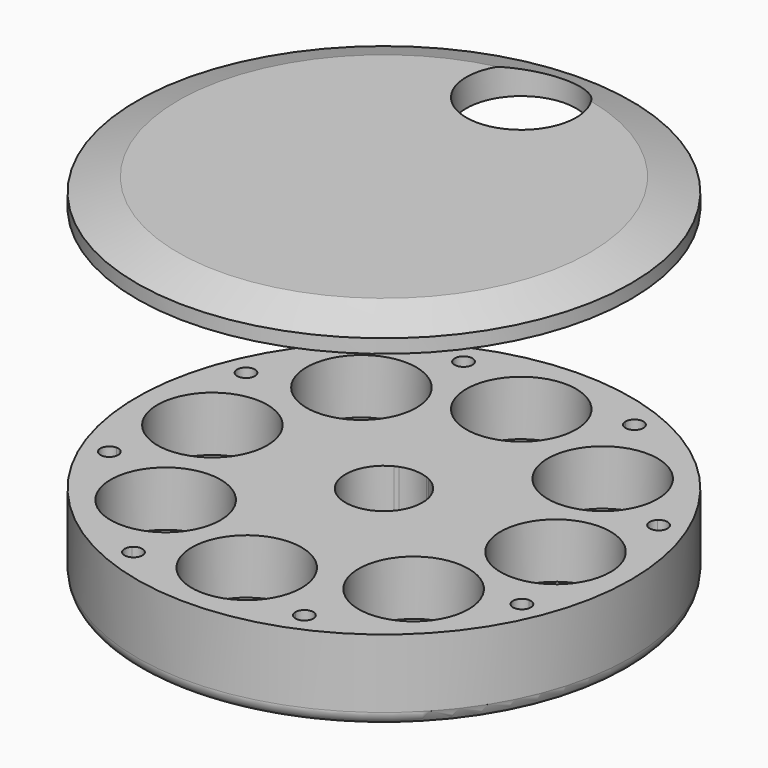
from build123d import *

# Parameters (mm, degrees)
F0_R       = 18
F0_R_2     = 4
F1_DEPTH   = 2
F2_DEPTH   = 4
F3_START   = 22
F3_DEPTH   = 2
F4_START   = 16
F4_DEPTH   = 8
F5_START   = 16
F5_DEPTH   = 2
F7_SIZE2   = 0.8
F7_SIZE    = 1.5
F7_2_SIZE2 = 0.8
F7_2_SIZE  = 1.5
F8_R       = 1
F10_START  = 3
F10_DEPTH  = 1
F11_START  = 21.4
F11_DEPTH  = 0.6
F12_R      = 0.5


# Not quite as in the source:
# - a fillet or chamfer that OpenCascade refuses, or shapes differently, is made with other operations: its cross-section is extruded or revolved along the edge and cut away or added


with BuildPart() as f1:
    # F0 (on Top) → F1 (new body)
    with BuildSketch(Plane.XY):
        Circle(F0_R)
        with Locations((-8.8177437266, -8.8598755958)):
            Circle(F0_R_2, mode=Mode.SUBTRACT)
        with Locations((0, -12.5)):
            Circle(F0_R_2, mode=Mode.SUBTRACT)
        with Locations((9.0546496307, -8.6176168437)):
            Circle(F0_R_2, mode=Mode.SUBTRACT)
        with Locations((-12.5, 0)):
            Circle(F0_R_2, mode=Mode.SUBTRACT)
        with Locations((-8.7692591217, 8.9078669981)):
            Circle(F0_R_2, mode=Mode.SUBTRACT)
        with BuildLine():
            Line((1, 3.25), (1, 3.0923292192))
            ThreePointArc((1, 3.0923292192), (1.5665779453, 2.8475135717), (2.0766559657, 2.5))
            Line((2.0766559657, 2.5), (3.25, 2.5))
            Line((3.25, 2.5), (3.25, 0))
            Line((3.25, 0), (3.25, -2.5))
            Line((3.25, -2.5), (2.0766559657, -2.5))
            ThreePointArc((2.0766559657, -2.5), (1.5665779453, -2.8475135717), (1, -3.0923292192))
            Line((1, -3.0923292192), (1, -3.25))
            Line((1, -3.25), (0, -3.25))
            Line((0, -3.25), (-1, -3.25))
            Line((-1, -3.25), (-1, -3.0923292192))
            ThreePointArc((-1, -3.0923292192), (-1.5665779453, -2.8475135717), (-2.0766559657, -2.5))
            Line((-2.0766559657, -2.5), (-3.25, -2.5))
            Line((-3.25, -2.5), (-3.25, 0))
            Line((-3.25, 0), (-3.25, 2.5))
            Line((-3.25, 2.5), (-2.0766559657, 2.5))
            ThreePointArc((-2.0766559657, 2.5), (-1.5665779453, 2.8475135717), (-1, 3.0923292192))
            Line((-1, 3.0923292192), (-1, 3.25))
            Line((-1, 3.25), (0, 3.25))
            Line((0, 3.25), (1, 3.25))
        make_face(mode=Mode.SUBTRACT)
        with Locations((8.9668709375, 8.7089164418)):
            Circle(F0_R_2, mode=Mode.SUBTRACT)
        with Locations((12.5, 0)):
            Circle(F0_R_2, mode=Mode.SUBTRACT)
        with Locations((0, 12.5)):
            Circle(F0_R_2, mode=Mode.SUBTRACT)
        with Locations((-8.7692591217, 8.9078669981)):
            Circle(F0_R_2)
        with Locations((0, 12.5)):
            Circle(F0_R_2)
        with Locations((12.5, 0)):
            Circle(F0_R_2)
        with Locations((9.0546496307, -8.6176168437)):
            Circle(F0_R_2)
        with Locations((0, -12.5)):
            Circle(F0_R_2)
        with Locations((8.9668709375, 8.7089164418)):
            Circle(F0_R_2)
        with Locations((-12.5, 0)):
            Circle(F0_R_2)
        with Locations((-8.8177437266, -8.8598755958)):
            Circle(F0_R_2)
        with BuildLine():
            Line((3.25, 2.5), (2.0766559657, 2.5))
            ThreePointArc((2.0766559657, 2.5), (2.942076808, 1.3808273084), (3.25, 0))
            Line((3.25, 0), (3.25, 2.5))
        make_face()
        with BuildLine():
            ThreePointArc((3.25, 0), (2.942076808, -1.3808273084), (2.0766559657, -2.5))
            Line((2.0766559657, -2.5), (3.25, -2.5))
            Line((3.25, -2.5), (3.25, 0))
        make_face()
        with BuildLine():
            Line((-3.25, -2.5), (-2.0766559657, -2.5))
            ThreePointArc((-2.0766559657, -2.5), (-2.942076808, -1.3808273084), (-3.25, 0))
            Line((-3.25, 0), (-3.25, -2.5))
        make_face()
        with BuildLine():
            ThreePointArc((-3.25, 0), (-2.942076808, 1.3808273084), (-2.0766559657, 2.5))
            Line((-2.0766559657, 2.5), (-3.25, 2.5))
            Line((-3.25, 2.5), (-3.25, 0))
        make_face()
        with BuildLine():
            Line((-1, 3.25), (-1, 3.0923292192))
            ThreePointArc((-1, 3.0923292192), (-0.5061768651, 3.2103403217), (0, 3.25))
            Line((0, 3.25), (-1, 3.25))
        make_face()
        with BuildLine():
            ThreePointArc((0, 3.25), (0.5061768651, 3.2103403217), (1, 3.0923292192))
            Line((1, 3.0923292192), (1, 3.25))
            Line((1, 3.25), (0, 3.25))
        make_face()
        with BuildLine():
            Line((1, -3.25), (1, -3.0923292192))
            ThreePointArc((1, -3.0923292192), (0.5061768651, -3.2103403217), (0, -3.25))
            Line((0, -3.25), (1, -3.25))
        make_face()
        with BuildLine():
            ThreePointArc((0, -3.25), (-0.5061768651, -3.2103403217), (-1, -3.0923292192))
            Line((-1, -3.0923292192), (-1, -3.25))
            Line((-1, -3.25), (0, -3.25))
        make_face()
    extrude(amount=-F1_DEPTH)

    # F0 (on Top) → F2 (join)
    with BuildSketch(Plane.XY):
        Circle(F0_R)
        with Locations((-8.8177437266, -8.8598755958)):
            Circle(F0_R_2, mode=Mode.SUBTRACT)
        with Locations((0, -12.5)):
            Circle(F0_R_2, mode=Mode.SUBTRACT)
        with Locations((9.0546496307, -8.6176168437)):
            Circle(F0_R_2, mode=Mode.SUBTRACT)
        with Locations((-12.5, 0)):
            Circle(F0_R_2, mode=Mode.SUBTRACT)
        with Locations((-8.7692591217, 8.9078669981)):
            Circle(F0_R_2, mode=Mode.SUBTRACT)
        with BuildLine():
            Line((1, 3.25), (1, 3.0923292192))
            ThreePointArc((1, 3.0923292192), (1.5665779453, 2.8475135717), (2.0766559657, 2.5))
            Line((2.0766559657, 2.5), (3.25, 2.5))
            Line((3.25, 2.5), (3.25, 0))
            Line((3.25, 0), (3.25, -2.5))
            Line((3.25, -2.5), (2.0766559657, -2.5))
            ThreePointArc((2.0766559657, -2.5), (1.5665779453, -2.8475135717), (1, -3.0923292192))
            Line((1, -3.0923292192), (1, -3.25))
            Line((1, -3.25), (0, -3.25))
            Line((0, -3.25), (-1, -3.25))
            Line((-1, -3.25), (-1, -3.0923292192))
            ThreePointArc((-1, -3.0923292192), (-1.5665779453, -2.8475135717), (-2.0766559657, -2.5))
            Line((-2.0766559657, -2.5), (-3.25, -2.5))
            Line((-3.25, -2.5), (-3.25, 0))
            Line((-3.25, 0), (-3.25, 2.5))
            Line((-3.25, 2.5), (-2.0766559657, 2.5))
            ThreePointArc((-2.0766559657, 2.5), (-1.5665779453, 2.8475135717), (-1, 3.0923292192))
            Line((-1, 3.0923292192), (-1, 3.25))
            Line((-1, 3.25), (0, 3.25))
            Line((0, 3.25), (1, 3.25))
        make_face(mode=Mode.SUBTRACT)
        with Locations((8.9668709375, 8.7089164418)):
            Circle(F0_R_2, mode=Mode.SUBTRACT)
        with Locations((12.5, 0)):
            Circle(F0_R_2, mode=Mode.SUBTRACT)
        with Locations((0, 12.5)):
            Circle(F0_R_2, mode=Mode.SUBTRACT)
        with BuildLine():
            ThreePointArc((-3.25, 0), (-2.942076808, 1.3808273084), (-2.0766559657, 2.5))
            Line((-2.0766559657, 2.5), (-3.25, 2.5))
            Line((-3.25, 2.5), (-3.25, 0))
        make_face()
        with BuildLine():
            ThreePointArc((-1, 2.6153393661), (0, 2.8), (1, 2.6153393661))
            Line((1, 2.6153393661), (1, 3.0923292192))
            ThreePointArc((1, 3.0923292192), (0.5061768651, 3.2103403217), (0, 3.25))
            ThreePointArc((0, 3.25), (-0.5061768651, 3.2103403217), (-1, 3.0923292192))
            Line((-1, 3.0923292192), (-1, 2.6153393661))
        make_face()
        with BuildLine():
            ThreePointArc((-1.2609520213, 2.5), (-1.1319460248, 2.560995548), (-1, 2.6153393661))
            Line((-1, 2.6153393661), (-1, 3.0923292192))
            ThreePointArc((-1, 3.0923292192), (-1.5665779453, 2.8475135717), (-2.0766559657, 2.5))
            Line((-2.0766559657, 2.5), (-1.2609520213, 2.5))
        make_face()
        with BuildLine():
            Line((1, 3.0923292192), (1, 2.6153393661))
            ThreePointArc((1, 2.6153393661), (1.1319460248, 2.560995548), (1.2609520213, 2.5))
            Line((1.2609520213, 2.5), (2.0766559657, 2.5))
            ThreePointArc((2.0766559657, 2.5), (1.5665779453, 2.8475135717), (1, 3.0923292192))
        make_face()
        with BuildLine():
            Line((2.0766559657, 2.5), (1.2609520213, 2.5))
            ThreePointArc((1.2609520213, 2.5), (2.3843935979, 1.4678784589), (2.8, 0))
            ThreePointArc((2.8, 0), (2.3843935979, -1.4678784589), (1.2609520213, -2.5))
            Line((1.2609520213, -2.5), (2.0766559657, -2.5))
            ThreePointArc((2.0766559657, -2.5), (2.942076808, -1.3808273084), (3.25, 0))
            ThreePointArc((3.25, 0), (2.942076808, 1.3808273084), (2.0766559657, 2.5))
        make_face()
        with BuildLine():
            ThreePointArc((1.2609520213, -2.5), (1.1319460248, -2.560995548), (1, -2.6153393661))
            Line((1, -2.6153393661), (1, -3.0923292192))
            ThreePointArc((1, -3.0923292192), (1.5665779453, -2.8475135717), (2.0766559657, -2.5))
            Line((2.0766559657, -2.5), (1.2609520213, -2.5))
        make_face()
        with BuildLine():
            ThreePointArc((3.25, 0), (2.942076808, -1.3808273084), (2.0766559657, -2.5))
            Line((2.0766559657, -2.5), (3.25, -2.5))
            Line((3.25, -2.5), (3.25, 0))
        make_face()
        with BuildLine():
            Line((3.25, 2.5), (2.0766559657, 2.5))
            ThreePointArc((2.0766559657, 2.5), (2.942076808, 1.3808273084), (3.25, 0))
            Line((3.25, 0), (3.25, 2.5))
        make_face()
        with BuildLine():
            Line((-3.25, -2.5), (-2.0766559657, -2.5))
            ThreePointArc((-2.0766559657, -2.5), (-2.942076808, -1.3808273084), (-3.25, 0))
            Line((-3.25, 0), (-3.25, -2.5))
        make_face()
        with BuildLine():
            Line((1, -3.0923292192), (1, -2.6153393661))
            ThreePointArc((1, -2.6153393661), (0, -2.8), (-1, -2.6153393661))
            Line((-1, -2.6153393661), (-1, -3.0923292192))
            ThreePointArc((-1, -3.0923292192), (-0.5061768651, -3.2103403217), (0, -3.25))
            ThreePointArc((0, -3.25), (0.5061768651, -3.2103403217), (1, -3.0923292192))
        make_face()
        with BuildLine():
            Line((-1, -3.0923292192), (-1, -2.6153393661))
            ThreePointArc((-1, -2.6153393661), (-1.1319460248, -2.560995548), (-1.2609520213, -2.5))
            Line((-1.2609520213, -2.5), (-2.0766559657, -2.5))
            ThreePointArc((-2.0766559657, -2.5), (-1.5665779453, -2.8475135717), (-1, -3.0923292192))
        make_face()
        with BuildLine():
            ThreePointArc((-1.2609520213, -2.5), (-2.8, 0), (-1.2609520213, 2.5))
            Line((-1.2609520213, 2.5), (-2.0766559657, 2.5))
            ThreePointArc((-2.0766559657, 2.5), (-2.942076808, 1.3808273084), (-3.25, 0))
            ThreePointArc((-3.25, 0), (-2.942076808, -1.3808273084), (-2.0766559657, -2.5))
            Line((-2.0766559657, -2.5), (-1.2609520213, -2.5))
        make_face()
        with BuildLine():
            ThreePointArc((0, -3.25), (-0.5061768651, -3.2103403217), (-1, -3.0923292192))
            Line((-1, -3.0923292192), (-1, -3.25))
            Line((-1, -3.25), (0, -3.25))
        make_face()
        with BuildLine():
            Line((1, -3.25), (1, -3.0923292192))
            ThreePointArc((1, -3.0923292192), (0.5061768651, -3.2103403217), (0, -3.25))
            Line((0, -3.25), (1, -3.25))
        make_face()
        with BuildLine():
            Line((-1, 3.25), (-1, 3.0923292192))
            ThreePointArc((-1, 3.0923292192), (-0.5061768651, 3.2103403217), (0, 3.25))
            Line((0, 3.25), (-1, 3.25))
        make_face()
        with BuildLine():
            ThreePointArc((0, 3.25), (0.5061768651, 3.2103403217), (1, 3.0923292192))
            Line((1, 3.0923292192), (1, 3.25))
            Line((1, 3.25), (0, 3.25))
        make_face()
    extrude(amount=F2_DEPTH)

    # F8
    f8_edges = [f1.edges().sort_by_distance(p)[0] for p in [
        (-18, 0, -2),
        (3.25, 0, -2),
    ]]
    fillet(f8_edges, radius=F8_R)

    # F9 (on Top) → F10 (cut)
    with BuildSketch(Plane.XY.offset(F10_START)):
        with BuildLine():
            Line((-6.6848586175, 14.5694375213), (-6.2252392097, 15.0290569291))
            Line((-6.2252392097, 15.0290569291), (-5.5752392097, 15.0290569291))
            ThreePointArc((-5.5752392097, 15.0290569291), (-6.4739834407, 15.6295786252), (-6.6848586175, 14.5694375213))
        make_face()
        with BuildLine():
            Line((-5.5752392097, 15.0290569291), (-6.2252392097, 15.0290569291))
            Line((-6.2252392097, 15.0290569291), (-6.6848586175, 14.5694375213))
            ThreePointArc((-6.6848586175, 14.5694375213), (-5.9764949787, 14.4285352329), (-5.5752392097, 15.0290569291))
        make_face()
        with BuildLine():
            ThreePointArc((-14.3790569291, 6.2252392097), (-14.4285352329, 6.4739834407), (-14.5694375213, 6.6848586175))
            Line((-14.5694375213, 6.6848586175), (-15.0290569291, 6.2252392097))
            Line((-15.0290569291, 6.2252392097), (-15.0290569291, 5.5752392097))
            ThreePointArc((-15.0290569291, 5.5752392097), (-14.5694375213, 5.7656198019), (-14.3790569291, 6.2252392097))
        make_face()
        with BuildLine():
            Line((-15.0290569291, 6.2252392097), (-14.5694375213, 6.6848586175))
            ThreePointArc((-14.5694375213, 6.6848586175), (-15.6295786252, 6.4739834407), (-15.0290569291, 5.5752392097))
            Line((-15.0290569291, 5.5752392097), (-15.0290569291, 6.2252392097))
        make_face()
        with BuildLine():
            Line((6.2252392097, 15.0290569291), (5.5752392097, 15.0290569291))
            ThreePointArc((5.5752392097, 15.0290569291), (5.9764949787, 14.4285352329), (6.6848586175, 14.5694375213))
            Line((6.6848586175, 14.5694375213), (6.2252392097, 15.0290569291))
        make_face()
        with BuildLine():
            ThreePointArc((6.8752392097, 15.0290569291), (6.2252392097, 15.6790569291), (5.5752392097, 15.0290569291))
            Line((5.5752392097, 15.0290569291), (6.2252392097, 15.0290569291))
            Line((6.2252392097, 15.0290569291), (6.6848586175, 14.5694375213))
            ThreePointArc((6.6848586175, 14.5694375213), (6.8257609058, 14.780312698), (6.8752392097, 15.0290569291))
        make_face()
        with BuildLine():
            Line((15.0290569291, 6.2252392097), (14.5694375213, 6.6848586175))
            ThreePointArc((14.5694375213, 6.6848586175), (14.4285352329, 5.9764949787), (15.0290569291, 5.5752392097))
            Line((15.0290569291, 5.5752392097), (15.0290569291, 6.2252392097))
        make_face()
        with BuildLine():
            ThreePointArc((15.6790569291, 6.2252392097), (15.2778011601, 6.8257609058), (14.5694375213, 6.6848586175))
            Line((14.5694375213, 6.6848586175), (15.0290569291, 6.2252392097))
            Line((15.0290569291, 6.2252392097), (15.0290569291, 5.5752392097))
            ThreePointArc((15.0290569291, 5.5752392097), (15.4886763368, 5.7656198019), (15.6790569291, 6.2252392097))
        make_face()
        with BuildLine():
            ThreePointArc((15.6790569291, -6.2252392097), (15.4886763368, -5.7656198019), (15.0290569291, -5.5752392097))
            Line((15.0290569291, -5.5752392097), (15.0290569291, -6.2252392097))
            Line((15.0290569291, -6.2252392097), (14.5694375213, -6.6848586175))
            ThreePointArc((14.5694375213, -6.6848586175), (15.2778011601, -6.8257609058), (15.6790569291, -6.2252392097))
        make_face()
        with BuildLine():
            Line((15.0290569291, -6.2252392097), (15.0290569291, -5.5752392097))
            ThreePointArc((15.0290569291, -5.5752392097), (14.4285352329, -5.9764949787), (14.5694375213, -6.6848586175))
            Line((14.5694375213, -6.6848586175), (15.0290569291, -6.2252392097))
        make_face()
        with BuildLine():
            ThreePointArc((6.8752392097, -15.0290569291), (6.8257609058, -14.780312698), (6.6848586175, -14.5694375213))
            Line((6.6848586175, -14.5694375213), (6.2252392097, -15.0290569291))
            Line((6.2252392097, -15.0290569291), (5.5752392097, -15.0290569291))
            ThreePointArc((5.5752392097, -15.0290569291), (6.2252392097, -15.6790569291), (6.8752392097, -15.0290569291))
        make_face()
        with BuildLine():
            Line((6.2252392097, -15.0290569291), (6.6848586175, -14.5694375213))
            ThreePointArc((6.6848586175, -14.5694375213), (5.9764949787, -14.4285352329), (5.5752392097, -15.0290569291))
            Line((5.5752392097, -15.0290569291), (6.2252392097, -15.0290569291))
        make_face()
        with BuildLine():
            ThreePointArc((-14.3790569291, -6.2252392097), (-14.5694375213, -5.7656198019), (-15.0290569291, -5.5752392097))
            Line((-15.0290569291, -5.5752392097), (-15.0290569291, -6.2252392097))
            Line((-15.0290569291, -6.2252392097), (-14.5694375213, -6.6848586175))
            ThreePointArc((-14.5694375213, -6.6848586175), (-14.4285352329, -6.4739834407), (-14.3790569291, -6.2252392097))
        make_face()
        with BuildLine():
            Line((-15.0290569291, -6.2252392097), (-15.0290569291, -5.5752392097))
            ThreePointArc((-15.0290569291, -5.5752392097), (-15.6295786252, -6.4739834407), (-14.5694375213, -6.6848586175))
            Line((-14.5694375213, -6.6848586175), (-15.0290569291, -6.2252392097))
        make_face()
        with BuildLine():
            ThreePointArc((-5.5752392097, -15.0290569291), (-5.9764949787, -14.4285352329), (-6.6848586175, -14.5694375213))
            Line((-6.6848586175, -14.5694375213), (-6.2252392097, -15.0290569291))
            Line((-6.2252392097, -15.0290569291), (-5.5752392097, -15.0290569291))
        make_face()
        with BuildLine():
            Line((-6.2252392097, -15.0290569291), (-6.6848586175, -14.5694375213))
            ThreePointArc((-6.6848586175, -14.5694375213), (-6.4739834407, -15.6295786252), (-5.5752392097, -15.0290569291))
            Line((-5.5752392097, -15.0290569291), (-6.2252392097, -15.0290569291))
        make_face()
    extrude(amount=F10_DEPTH, mode=Mode.SUBTRACT)


with BuildPart() as f3:
    # F0 (on Top) → F3 (new body)
    with BuildSketch(Plane.XY.offset(F3_START)):
        Circle(F0_R)
        with Locations((-8.8177437266, -8.8598755958)):
            Circle(F0_R_2, mode=Mode.SUBTRACT)
        with Locations((0, -12.5)):
            Circle(F0_R_2, mode=Mode.SUBTRACT)
        with Locations((9.0546496307, -8.6176168437)):
            Circle(F0_R_2, mode=Mode.SUBTRACT)
        with Locations((-12.5, 0)):
            Circle(F0_R_2, mode=Mode.SUBTRACT)
        with Locations((-8.7692591217, 8.9078669981)):
            Circle(F0_R_2, mode=Mode.SUBTRACT)
        with BuildLine():
            Line((1, 3.25), (1, 3.0923292192))
            ThreePointArc((1, 3.0923292192), (1.5665779453, 2.8475135717), (2.0766559657, 2.5))
            Line((2.0766559657, 2.5), (3.25, 2.5))
            Line((3.25, 2.5), (3.25, 0))
            Line((3.25, 0), (3.25, -2.5))
            Line((3.25, -2.5), (2.0766559657, -2.5))
            ThreePointArc((2.0766559657, -2.5), (1.5665779453, -2.8475135717), (1, -3.0923292192))
            Line((1, -3.0923292192), (1, -3.25))
            Line((1, -3.25), (0, -3.25))
            Line((0, -3.25), (-1, -3.25))
            Line((-1, -3.25), (-1, -3.0923292192))
            ThreePointArc((-1, -3.0923292192), (-1.5665779453, -2.8475135717), (-2.0766559657, -2.5))
            Line((-2.0766559657, -2.5), (-3.25, -2.5))
            Line((-3.25, -2.5), (-3.25, 0))
            Line((-3.25, 0), (-3.25, 2.5))
            Line((-3.25, 2.5), (-2.0766559657, 2.5))
            ThreePointArc((-2.0766559657, 2.5), (-1.5665779453, 2.8475135717), (-1, 3.0923292192))
            Line((-1, 3.0923292192), (-1, 3.25))
            Line((-1, 3.25), (0, 3.25))
            Line((0, 3.25), (1, 3.25))
        make_face(mode=Mode.SUBTRACT)
        with Locations((8.9668709375, 8.7089164418)):
            Circle(F0_R_2, mode=Mode.SUBTRACT)
        with Locations((12.5, 0)):
            Circle(F0_R_2, mode=Mode.SUBTRACT)
        with Locations((0, 12.5)):
            Circle(F0_R_2, mode=Mode.SUBTRACT)
        with Locations((-8.8177437266, -8.8598755958)):
            Circle(F0_R_2)
        with Locations((-12.5, 0)):
            Circle(F0_R_2)
        with Locations((-8.7692591217, 8.9078669981)):
            Circle(F0_R_2)
        with Locations((8.9668709375, 8.7089164418)):
            Circle(F0_R_2)
        with Locations((12.5, 0)):
            Circle(F0_R_2)
        with Locations((9.0546496307, -8.6176168437)):
            Circle(F0_R_2)
        with Locations((0, -12.5)):
            Circle(F0_R_2)
        with BuildLine():
            ThreePointArc((-3.25, 0), (-2.942076808, 1.3808273084), (-2.0766559657, 2.5))
            Line((-2.0766559657, 2.5), (-3.25, 2.5))
            Line((-3.25, 2.5), (-3.25, 0))
        make_face()
        with BuildLine():
            Line((-3.25, -2.5), (-2.0766559657, -2.5))
            ThreePointArc((-2.0766559657, -2.5), (-2.942076808, -1.3808273084), (-3.25, 0))
            Line((-3.25, 0), (-3.25, -2.5))
        make_face()
        with BuildLine():
            ThreePointArc((0, -3.25), (-0.5061768651, -3.2103403217), (-1, -3.0923292192))
            Line((-1, -3.0923292192), (-1, -3.25))
            Line((-1, -3.25), (0, -3.25))
        make_face()
        with BuildLine():
            Line((1, -3.25), (1, -3.0923292192))
            ThreePointArc((1, -3.0923292192), (0.5061768651, -3.2103403217), (0, -3.25))
            Line((0, -3.25), (1, -3.25))
        make_face()
        with BuildLine():
            ThreePointArc((3.25, 0), (2.942076808, -1.3808273084), (2.0766559657, -2.5))
            Line((2.0766559657, -2.5), (3.25, -2.5))
            Line((3.25, -2.5), (3.25, 0))
        make_face()
        with BuildLine():
            Line((3.25, 2.5), (2.0766559657, 2.5))
            ThreePointArc((2.0766559657, 2.5), (2.942076808, 1.3808273084), (3.25, 0))
            Line((3.25, 0), (3.25, 2.5))
        make_face()
        with BuildLine():
            ThreePointArc((0, 3.25), (0.5061768651, 3.2103403217), (1, 3.0923292192))
            Line((1, 3.0923292192), (1, 3.25))
            Line((1, 3.25), (0, 3.25))
        make_face()
        with BuildLine():
            Line((-1, 3.25), (-1, 3.0923292192))
            ThreePointArc((-1, 3.0923292192), (-0.5061768651, 3.2103403217), (0, 3.25))
            Line((0, 3.25), (-1, 3.25))
        make_face()
        with BuildLine():
            ThreePointArc((-1, 2.6153393661), (0, 2.8), (1, 2.6153393661))
            Line((1, 2.6153393661), (1, 3.0923292192))
            ThreePointArc((1, 3.0923292192), (0.5061768651, 3.2103403217), (0, 3.25))
            ThreePointArc((0, 3.25), (-0.5061768651, 3.2103403217), (-1, 3.0923292192))
            Line((-1, 3.0923292192), (-1, 2.6153393661))
        make_face()
        with BuildLine():
            ThreePointArc((-1.2609520213, 2.5), (-1.1319460248, 2.560995548), (-1, 2.6153393661))
            Line((-1, 2.6153393661), (-1, 3.0923292192))
            ThreePointArc((-1, 3.0923292192), (-1.5665779453, 2.8475135717), (-2.0766559657, 2.5))
            Line((-2.0766559657, 2.5), (-1.2609520213, 2.5))
        make_face()
        with BuildLine():
            Line((2.0766559657, 2.5), (1.2609520213, 2.5))
            ThreePointArc((1.2609520213, 2.5), (2.3843935979, 1.4678784589), (2.8, 0))
            ThreePointArc((2.8, 0), (2.3843935979, -1.4678784589), (1.2609520213, -2.5))
            Line((1.2609520213, -2.5), (2.0766559657, -2.5))
            ThreePointArc((2.0766559657, -2.5), (2.942076808, -1.3808273084), (3.25, 0))
            ThreePointArc((3.25, 0), (2.942076808, 1.3808273084), (2.0766559657, 2.5))
        make_face()
        with BuildLine():
            ThreePointArc((1.2609520213, -2.5), (1.1319460248, -2.560995548), (1, -2.6153393661))
            Line((1, -2.6153393661), (1, -3.0923292192))
            ThreePointArc((1, -3.0923292192), (1.5665779453, -2.8475135717), (2.0766559657, -2.5))
            Line((2.0766559657, -2.5), (1.2609520213, -2.5))
        make_face()
        with BuildLine():
            Line((1, -3.0923292192), (1, -2.6153393661))
            ThreePointArc((1, -2.6153393661), (0, -2.8), (-1, -2.6153393661))
            Line((-1, -2.6153393661), (-1, -3.0923292192))
            ThreePointArc((-1, -3.0923292192), (-0.5061768651, -3.2103403217), (0, -3.25))
            ThreePointArc((0, -3.25), (0.5061768651, -3.2103403217), (1, -3.0923292192))
        make_face()
        with BuildLine():
            Line((-1, -3.0923292192), (-1, -2.6153393661))
            ThreePointArc((-1, -2.6153393661), (-1.1319460248, -2.560995548), (-1.2609520213, -2.5))
            Line((-1.2609520213, -2.5), (-2.0766559657, -2.5))
            ThreePointArc((-2.0766559657, -2.5), (-1.5665779453, -2.8475135717), (-1, -3.0923292192))
        make_face()
        with BuildLine():
            ThreePointArc((-1.2609520213, -2.5), (-2.8, 0), (-1.2609520213, 2.5))
            Line((-1.2609520213, 2.5), (-2.0766559657, 2.5))
            ThreePointArc((-2.0766559657, 2.5), (-2.942076808, 1.3808273084), (-3.25, 0))
            ThreePointArc((-3.25, 0), (-2.942076808, -1.3808273084), (-2.0766559657, -2.5))
            Line((-2.0766559657, -2.5), (-1.2609520213, -2.5))
        make_face()
        with BuildLine():
            Line((-1, -2.6153393661), (-1, -2.5))
            Line((-1, -2.5), (-1.2609520213, -2.5))
            ThreePointArc((-1.2609520213, -2.5), (-1.1319460248, -2.560995548), (-1, -2.6153393661))
        make_face()
        with BuildLine():
            Line((1, -2.5), (0, -2.5))
            Line((0, -2.5), (-1, -2.5))
            Line((-1, -2.5), (-1, -2.6153393661))
            ThreePointArc((-1, -2.6153393661), (0, -2.8), (1, -2.6153393661))
            Line((1, -2.6153393661), (1, -2.5))
        make_face()
        with BuildLine():
            Line((1.2609520213, -2.5), (1, -2.5))
            Line((1, -2.5), (1, -2.6153393661))
            ThreePointArc((1, -2.6153393661), (1.1319460248, -2.560995548), (1.2609520213, -2.5))
        make_face()
        with BuildLine():
            ThreePointArc((1, 2.2912878475), (2.0916500663, 1.3693063938), (2.5, 0))
            ThreePointArc((2.5, 0), (2.0916500663, -1.3693063938), (1, -2.2912878475))
            Line((1, -2.2912878475), (1, -2.5))
            Line((1, -2.5), (1.2609520213, -2.5))
            ThreePointArc((1.2609520213, -2.5), (2.3843935979, -1.4678784589), (2.8, 0))
            ThreePointArc((2.8, 0), (2.3843935979, 1.4678784589), (1.2609520213, 2.5))
            Line((1.2609520213, 2.5), (1, 2.5))
            Line((1, 2.5), (1, 2.2912878475))
        make_face()
        with BuildLine():
            Line((1, -2.5), (1, -2.2912878475))
            ThreePointArc((1, -2.2912878475), (0.5107741092, -2.4472657823), (0, -2.5))
            Line((0, -2.5), (1, -2.5))
        make_face()
        with BuildLine():
            Line((-1, -2.5), (0, -2.5))
            ThreePointArc((0, -2.5), (-0.5107741092, -2.4472657823), (-1, -2.2912878475))
            Line((-1, -2.2912878475), (-1, -2.5))
        make_face()
        with BuildLine():
            ThreePointArc((-1, -2.2912878475), (-2.5, 0), (-1, 2.2912878475))
            Line((-1, 2.2912878475), (-1, 2.5))
            Line((-1, 2.5), (-1.2609520213, 2.5))
            ThreePointArc((-1.2609520213, 2.5), (-2.8, 0), (-1.2609520213, -2.5))
            Line((-1.2609520213, -2.5), (-1, -2.5))
            Line((-1, -2.5), (-1, -2.2912878475))
        make_face()
        with BuildLine():
            ThreePointArc((-1, 2.2912878475), (-0.5107741092, 2.4472657823), (0, 2.5))
            Line((0, 2.5), (-1, 2.5))
            Line((-1, 2.5), (-1, 2.2912878475))
        make_face()
        with BuildLine():
            Line((-1.2609520213, 2.5), (-1, 2.5))
            Line((-1, 2.5), (-1, 2.6153393661))
            ThreePointArc((-1, 2.6153393661), (-1.1319460248, 2.560995548), (-1.2609520213, 2.5))
        make_face()
        with BuildLine():
            Line((1, 3.0923292192), (1, 2.6153393661))
            ThreePointArc((1, 2.6153393661), (1.1319460248, 2.560995548), (1.2609520213, 2.5))
            Line((1.2609520213, 2.5), (2.0766559657, 2.5))
            ThreePointArc((2.0766559657, 2.5), (1.5665779453, 2.8475135717), (1, 3.0923292192))
        make_face()
        with BuildLine():
            Line((1, 2.6153393661), (1, 2.5))
            Line((1, 2.5), (1.2609520213, 2.5))
            ThreePointArc((1.2609520213, 2.5), (1.1319460248, 2.560995548), (1, 2.6153393661))
        make_face()
        with BuildLine():
            Line((-1, 2.5), (0, 2.5))
            Line((0, 2.5), (1, 2.5))
            Line((1, 2.5), (1, 2.6153393661))
            ThreePointArc((1, 2.6153393661), (0, 2.8), (-1, 2.6153393661))
            Line((-1, 2.6153393661), (-1, 2.5))
        make_face()
        with BuildLine():
            ThreePointArc((0, 2.5), (0.5107741092, 2.4472657823), (1, 2.2912878475))
            Line((1, 2.2912878475), (1, 2.5))
            Line((1, 2.5), (0, 2.5))
        make_face()
        with BuildLine():
            ThreePointArc((1, -2.2912878475), (2.0916500663, -1.3693063938), (2.5, 0))
            ThreePointArc((2.5, 0), (2.0916500663, 1.3693063938), (1, 2.2912878475))
            Line((1, 2.2912878475), (1, -2.2912878475))
        make_face()
        with BuildLine():
            Line((1, -2.2912878475), (1, 2.2912878475))
            ThreePointArc((1, 2.2912878475), (0.5107741092, 2.4472657823), (0, 2.5))
            ThreePointArc((0, 2.5), (-0.5107741092, 2.4472657823), (-1, 2.2912878475))
            Line((-1, 2.2912878475), (-1, -2.2912878475))
            ThreePointArc((-1, -2.2912878475), (-0.5107741092, -2.4472657823), (0, -2.5))
            ThreePointArc((0, -2.5), (0.5107741092, -2.4472657823), (1, -2.2912878475))
        make_face()
        with BuildLine():
            Line((-1, -2.2912878475), (-1, 2.2912878475))
            ThreePointArc((-1, 2.2912878475), (-2.5, 0), (-1, -2.2912878475))
        make_face()
    extrude(amount=F3_DEPTH)

    # F0 (on Top) → F4 (join)
    with BuildSketch(Plane.XY.offset(F4_START)):
        with BuildLine():
            ThreePointArc((1, -2.2912878475), (2.0916500663, -1.3693063938), (2.5, 0))
            ThreePointArc((2.5, 0), (2.0916500663, 1.3693063938), (1, 2.2912878475))
            Line((1, 2.2912878475), (1, -2.2912878475))
        make_face()
        with BuildLine():
            Line((-1, -2.2912878475), (-1, 2.2912878475))
            ThreePointArc((-1, 2.2912878475), (-2.5, 0), (-1, -2.2912878475))
        make_face()
    extrude(amount=F4_DEPTH)

    # F0 (on Top) → F5 (join)
    with BuildSketch(Plane.XY.offset(F5_START)):
        with BuildLine():
            ThreePointArc((1, 2.2912878475), (2.0916500663, 1.3693063938), (2.5, 0))
            ThreePointArc((2.5, 0), (2.0916500663, -1.3693063938), (1, -2.2912878475))
            Line((1, -2.2912878475), (1, -2.5))
            Line((1, -2.5), (1.2609520213, -2.5))
            ThreePointArc((1.2609520213, -2.5), (2.3843935979, -1.4678784589), (2.8, 0))
            ThreePointArc((2.8, 0), (2.3843935979, 1.4678784589), (1.2609520213, 2.5))
            Line((1.2609520213, 2.5), (1, 2.5))
            Line((1, 2.5), (1, 2.2912878475))
        make_face()
        with BuildLine():
            ThreePointArc((-1, -2.2912878475), (-2.5, 0), (-1, 2.2912878475))
            Line((-1, 2.2912878475), (-1, 2.5))
            Line((-1, 2.5), (-1.2609520213, 2.5))
            ThreePointArc((-1.2609520213, 2.5), (-2.8, 0), (-1.2609520213, -2.5))
            Line((-1.2609520213, -2.5), (-1, -2.5))
            Line((-1, -2.5), (-1, -2.2912878475))
        make_face()
    extrude(amount=F5_DEPTH)

    # F6: chamfer of 3 x 1 on 1 edges, made by hand

    # F6_s1 → F6_t2 (revolve, cut)
    with BuildSketch(Plane.XZ):
        Polygon((18, 23), (15, 24), (18, 24), align=None)
    revolve(axis=Axis((0, 0, 24), (0, 0, 1)), mode=Mode.SUBTRACT)

    # F7
    f7_edges = [f3.edges().sort_by_distance(p)[0] for p in [
        (-2.8, 0, 16),
    ]]
    f7_side = f3.faces().sort_by_distance((-2.8, 0, 17))[0]
    chamfer(f7_edges, length=F7_SIZE, length2=F7_SIZE2, reference=f7_side)

    # F7#2
    f7_2_edges = [f3.edges().sort_by_distance(p)[0] for p in [
        (2.8, 0, 16),
    ]]
    f7_2_side = f3.faces().sort_by_distance((2.8, 0, 17))[0]
    chamfer(f7_2_edges, length=F7_2_SIZE, length2=F7_2_SIZE2, reference=f7_2_side)

    # F9 (on Top) → F11 (join)
    with BuildSketch(Plane.XY.offset(F11_START)):
        with BuildLine():
            ThreePointArc((6.8752392097, -15.0290569291), (6.8257609058, -14.780312698), (6.6848586175, -14.5694375213))
            Line((6.6848586175, -14.5694375213), (6.2252392097, -15.0290569291))
            Line((6.2252392097, -15.0290569291), (5.5752392097, -15.0290569291))
            ThreePointArc((5.5752392097, -15.0290569291), (6.2252392097, -15.6790569291), (6.8752392097, -15.0290569291))
        make_face()
        with BuildLine():
            Line((6.2252392097, -15.0290569291), (6.6848586175, -14.5694375213))
            ThreePointArc((6.6848586175, -14.5694375213), (5.9764949787, -14.4285352329), (5.5752392097, -15.0290569291))
            Line((5.5752392097, -15.0290569291), (6.2252392097, -15.0290569291))
        make_face()
        with BuildLine():
            Line((-6.6848586175, 14.5694375213), (-6.2252392097, 15.0290569291))
            Line((-6.2252392097, 15.0290569291), (-5.5752392097, 15.0290569291))
            ThreePointArc((-5.5752392097, 15.0290569291), (-6.4739834407, 15.6295786252), (-6.6848586175, 14.5694375213))
        make_face()
        with BuildLine():
            Line((-5.5752392097, 15.0290569291), (-6.2252392097, 15.0290569291))
            Line((-6.2252392097, 15.0290569291), (-6.6848586175, 14.5694375213))
            ThreePointArc((-6.6848586175, 14.5694375213), (-5.9764949787, 14.4285352329), (-5.5752392097, 15.0290569291))
        make_face()
    extrude(amount=F11_DEPTH)

    # F12
    f12_edges = [f3.edges().sort_by_distance(p)[0] for p in [
        (5.575239, -15.029057, 21.4),
        (-5.76562, 15.488676, 21.4),
    ]]
    fillet(f12_edges, radius=F12_R)


solid = Compound([f1.part, f3.part])
